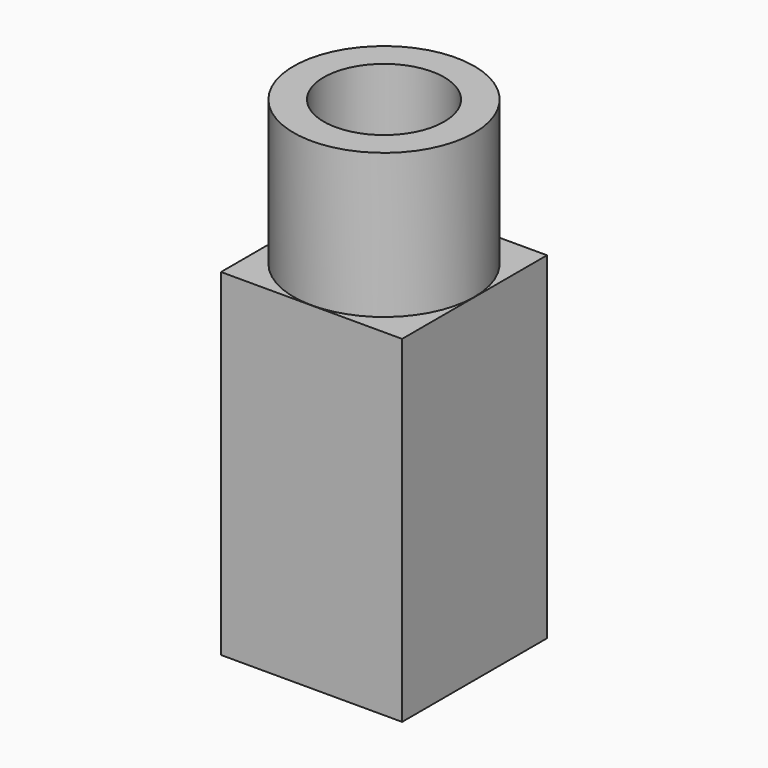
from build123d import *

# Parameters (mm, degrees)
F0_R     = 2.38125
F1_DEPTH = 6.35
F2_R     = 1.5875
F3_DEPTH = 6.35
F4_W     = 4.7752
F4_H     = 4.7752
F4_R     = 2.38125
F5_DEPTH = 2.54
F6_DEPTH = 6.35


with BuildPart() as f1:
    # F0 (on Top) → F1 (new body)
    with BuildSketch(Plane.XY):
        Circle(F0_R)
    extrude(amount=F1_DEPTH)

    # F2 (on face) → F3 (cut)
    with BuildSketch(Plane.XY.offset(6.35)):
        Circle(F2_R)
    extrude(amount=-F3_DEPTH, mode=Mode.SUBTRACT)

    # F4 (on face) → F5 (join)
    with BuildSketch(Plane(origin=(0, 0, 0), x_dir=(1, 0, 0), z_dir=(0, 0, -1))):
        Rectangle(F4_W, F4_H)
        Circle(F4_R, mode=Mode.SUBTRACT)
    extrude(amount=-F5_DEPTH)

    # F6 (add): a face of the model
    f6_faces = [f1.faces().sort_by_distance(p)[0] for p in [
        (-2.320068474, 0, 0),
    ]]
    extrude(f6_faces, amount=F6_DEPTH)


solid = f1.part
